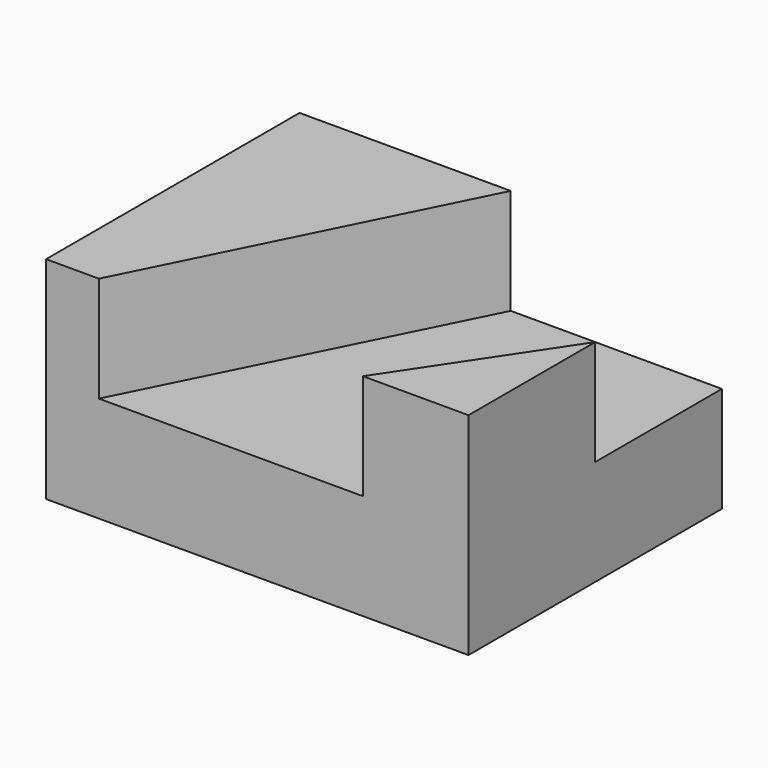
from build123d import *

# Parameters (mm, degrees)
F0_W     = 50.8
F0_H     = 25.4
F1_DEPTH = 38.1
F3_DEPTH = 12.7


# Not quite as in the source:
# - a length typed as a fraction of an inch, garbled in the dataset ("3 / 203.2 mm" for 3/8 in), is restored


with BuildPart() as f1:
    # F0 (on Front) → F1 (new body)
    with BuildSketch(Plane.XZ):
        with Locations((-40.7616753732, 12.7)):
            Rectangle(F0_W, F0_H)
    extrude(amount=F1_DEPTH)

    # F2 (on face) → F3 (cut)
    with BuildSketch(Plane.XY.offset(25.4)):
        Polygon((-15.3616753732, 0), (-40.7616753732, 0), (-59.8116753732, -38.1), (-28.0616753732, -38.1), (-15.3616753732, -19.05), align=None)
    extrude(amount=-F3_DEPTH, mode=Mode.SUBTRACT)


solid = f1.part
